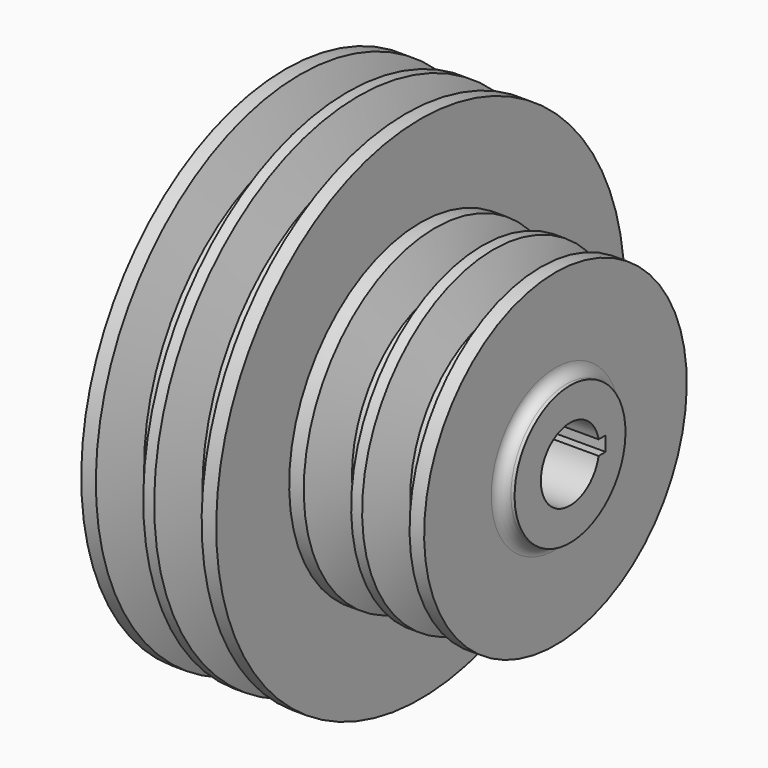
from build123d import *

# Parameters (mm, degrees)
F3_DEPTH = 78.001


with BuildPart() as f1:
    # F0 (on Front) → F1 (revolve)
    with BuildSketch(Plane.XZ):
        with BuildLine():
            Line((-27, 10), (41, 10))
            Line((41, 10), (41, 19))
            Line((41, 19), (40, 19))
            ThreePointArc((40, 19), (37.8786796564, 19.8786796564), (37, 22))
            Line((37, 22), (37, 45))
            Line((37, 45), (33, 45))
            Line((33, 45), (29.3465183566, 33.05))
            Line((29.3465183566, 33.05), (23.6534816434, 33.05))
            Line((23.6534816434, 33.05), (20, 45))
            Line((20, 45), (17, 45))
            Line((17, 45), (13.3465183566, 33.05))
            Line((13.3465183566, 33.05), (7.6534816434, 33.05))
            Line((7.6534816434, 33.05), (4, 45))
            Line((4, 45), (0, 45))
            Line((0, 45), (0, 70))
            Line((0, 70), (-4, 70))
            Line((-4, 70), (-7.6534816434, 58.05))
            Line((-7.6534816434, 58.05), (-13.3465183566, 58.05))
            Line((-13.3465183566, 58.05), (-17, 70))
            Line((-17, 70), (-20, 70))
            Line((-20, 70), (-23.6534816434, 58.05))
            Line((-23.6534816434, 58.05), (-29.3465183566, 58.05))
            Line((-29.3465183566, 58.05), (-33, 70))
            Line((-33, 70), (-37, 70))
            Line((-37, 70), (-37, 35))
            Line((-37, 35), (-32, 35))
            ThreePointArc((-32, 35), (-28.4644660941, 33.5355339059), (-27, 30))
            Line((-27, 30), (-27, 10))
        make_face()
    revolve(axis=Axis((1.6295525322, 0, 0), (1, 0, 0)))

    # F2 (on face) → F3 (cut, through all)
    with BuildSketch(Plane.YZ.offset(41)):
        with BuildLine():
            ThreePointArc((9.7979589711, 2), (-10, 0), (9.7979589711, -2))
            ThreePointArc((9.7979589711, -2), (9.9493615301, -1.0050896201), (10, 0))
            ThreePointArc((10, 0), (9.9493615301, 1.0050896201), (9.7979589711, 2))
        make_face()
        with BuildLine():
            ThreePointArc((10, 0), (9.9493615301, -1.0050896201), (9.7979589711, -2))
            Line((9.7979589711, -2), (12.2, -2))
            Line((12.2, -2), (12.2, 2))
            Line((12.2, 2), (9.7979589711, 2))
            ThreePointArc((9.7979589711, 2), (9.9493615301, 1.0050896201), (10, 0))
        make_face()
    extrude(amount=-F3_DEPTH, mode=Mode.SUBTRACT)


solid = f1.part
